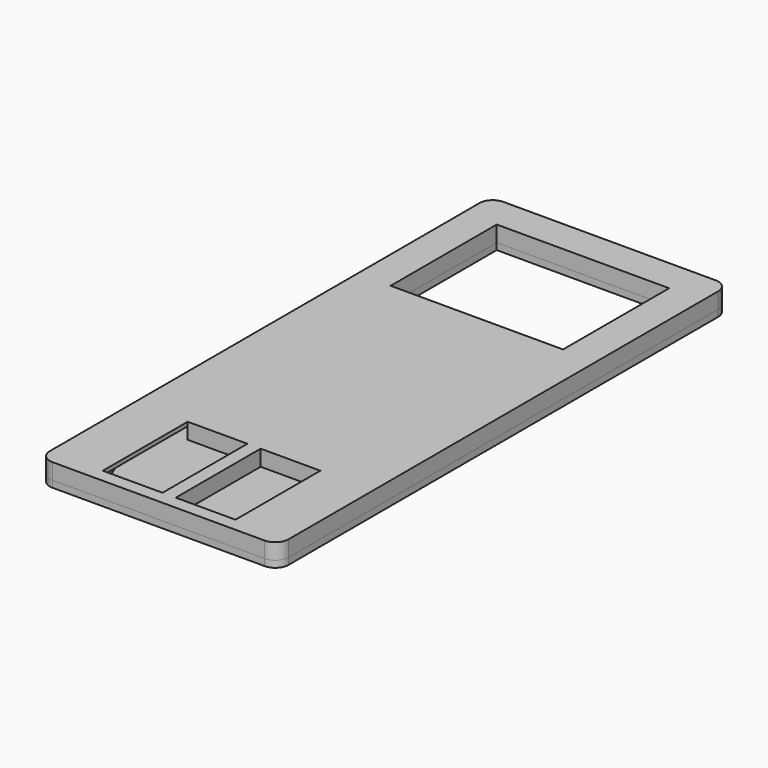
from build123d import *

# Parameters (mm, degrees)
F0_W      = 36
F0_H      = 30
F0_W_2    = 26
F0_H_2    = 20
F0_H_3    = 37
F0_H_4    = 18
F1_DEPTH  = 2.4
F2_W      = 34
F2_H      = 83
F2_W_2    = 28
F2_H_2    = 22
F3_DEPTH  = 1.8
F4_W      = 36
F4_H      = 1
F5_DEPTH  = 85
F8_DEPTH  = 1.8
F6_R      = 1
F9_DEPTH  = 3
F6_W      = 26
F6_H      = 20
F11_DEPTH = 25
F12_R     = 2
F12_2_R   = 2
F10_W     = 9
F10_H     = 16
F13_DEPTH = 3


# Not quite as in the source:
# - a feature names something its author has since deleted; it is built from what else it names


with BuildPart() as f1:
    # F0 (on Top) → F1 (new body)
    with BuildSketch(Plane.XY):
        Rectangle(F0_W, F0_H)
        Rectangle(F0_W_2, F0_H_2, mode=Mode.SUBTRACT)
        with Locations((0, -33.5)):
            Rectangle(F0_W, F0_H_3)
        with Locations((0, -61)):
            Rectangle(F0_W, F0_H_4)
    extrude(amount=F1_DEPTH)

    # F2 (on face) → F3 (cut)
    with BuildSketch(Plane(origin=(0, 0, 0), x_dir=(1, 0, 0), z_dir=(0, 0, -1))):
        with Locations((0, 27.5)):
            Rectangle(F2_W, F2_H)
        Rectangle(F2_W_2, F2_H_2, mode=Mode.SUBTRACT)
    extrude(amount=-F3_DEPTH, mode=Mode.SUBTRACT)

    # F7 (on face) → F8 (join, through all)
    with BuildSketch(Plane(origin=(0, 0, 1.8), x_dir=(1, 0, 0), z_dir=(0, 0, -1))):
        Polygon((-10, 14), (0, 14), (10, 14), (10, 52), (1, 52), (0, 52), (-1, 52), (-10, 52), align=None)
        Polygon((-1, 68.013086915), (-1, 52), (0, 52), (1, 52), (1, 68.013086915), align=None)
        Polygon((-10.0040324032, 68.013086915), (-1, 68.013086915), (1, 68.013086915), (10.0048035383, 68.013086915), (17, 51.7664179206), (17, 69), (-17, 69), (-17, 53.814060986), (-17, 51.7814494669), align=None)
    extrude(amount=F8_DEPTH)

    # F12
    f12_edges = [f1.edges().sort_by_distance(p)[0] for p in [
        (18, 15, 1.2),
        (18, -70, 1.2),
        (-18, -70, 1.2),
        (-18, 15, 1.2),
    ]]
    fillet(f12_edges, radius=F12_R)

    # F10 (on face) → F13 (cut)
    with BuildSketch(Plane.XY.offset(2.4)):
        with Locations((5.5, -60)):
            Rectangle(F10_W, F10_H)
        with Locations((-5.5, -60)):
            Rectangle(F10_W, F10_H)
    extrude(amount=-F13_DEPTH, mode=Mode.SUBTRACT)


with BuildPart() as f5:
    # F4 (on face) → F5 (new body, through all)
    with BuildSketch(Plane.XZ.offset(70)):
        with Locations((0, -0.5)):
            Rectangle(F4_W, F4_H)
    extrude(amount=-F5_DEPTH)

    # F6 (on face) → F9 (cut)
    with BuildSketch(Plane(origin=(0, 0, -1), x_dir=(1, 0, 0), z_dir=(0, 0, -1))):
        with Locations((-15, -12)):
            Circle(F6_R)
        with Locations((-9, -12)):
            Circle(F6_R)
        with Locations((-3, -12)):
            Circle(F6_R)
        with Locations((3, -12)):
            Circle(F6_R)
        with Locations((9, -12)):
            Circle(F6_R)
        with Locations((15, -12)):
            Circle(F6_R)
        with Locations((15, -6)):
            Circle(F6_R)
        with Locations((15, 0)):
            Circle(F6_R)
        with Locations((15, 6)):
            Circle(F6_R)
        with Locations((15, 12)):
            Circle(F6_R)
        with Locations((9, 12)):
            Circle(F6_R)
        with Locations((3, 12)):
            Circle(F6_R)
        with Locations((-3, 12)):
            Circle(F6_R)
        with Locations((-9, 12)):
            Circle(F6_R)
        with Locations((-15, 12)):
            Circle(F6_R)
        with Locations((-15, 6.6)):
            Circle(F6_R)
        with Locations((-15, 1.2)):
            Circle(F6_R)
        with Locations((-15, -4.2)):
            Circle(F6_R)
    extrude(amount=-F9_DEPTH, mode=Mode.SUBTRACT)

    # F6 (on face) → F11 (cut)
    with BuildSketch(Plane(origin=(0, 0, -1), x_dir=(1, 0, 0), z_dir=(0, 0, -1))):
        Rectangle(F6_W, F6_H)
    extrude(amount=-F11_DEPTH, mode=Mode.SUBTRACT)

    # F12#2
    f12_2_edges = [f5.edges().sort_by_distance(p)[0] for p in [
        (18, 15, -0.5),
        (18, -70, -0.5),
        (-18, -70, -0.5),
        (-18, 15, -0.5),
    ]]
    fillet(f12_2_edges, radius=F12_2_R)


solid = Compound([f1.part, f5.part])
